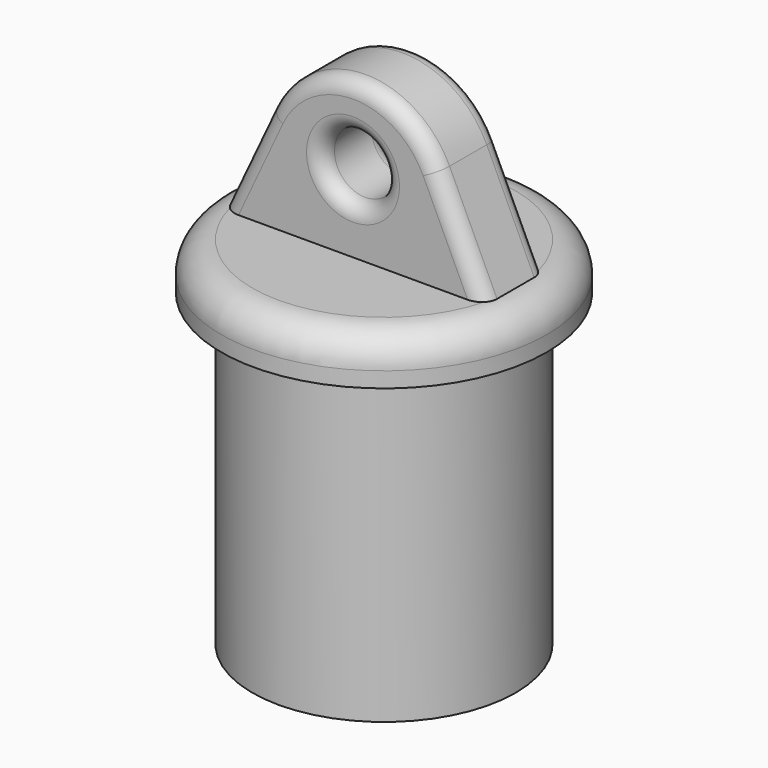
from build123d import *

# Parameters (mm, degrees)
F0_R          = 10.5
F1_DEPTH      = 3
F2_R          = 2
F3_R          = 7
F4_DEPTH      = 0.5
F5_W          = 1.5
F5_H          = 20
F7_R          = 2
F8_DEPTH      = 2.5
F8_DEPTH_BACK = 2.5
F9_T8_DEPTH   = 9.7284161474
F9_T13_DEPTH  = 9.7284161474
F9_T16_ANGLE  = 129.7914851202
F9_T20_DEPTH  = 9.7284161474
F9_T23_ANGLE  = 129.7914851202
F9_T27_DEPTH  = 9.7284161474


# Not quite as in the source:
# - a fillet or chamfer that OpenCascade refuses, or shapes differently, is made with other operations: its cross-section is extruded or revolved along the edge and cut away or added


with BuildPart() as f1:
    # F0 (on Top) → F1 (new body)
    with BuildSketch(Plane.XY):
        Circle(F0_R)
    extrude(amount=F1_DEPTH)

    # F2
    f2_edges = [f1.edges().sort_by_distance(p)[0] for p in [
        (-10.5, 0, 3),
    ]]
    fillet(f2_edges, radius=F2_R)

    # F3 (on face) → F4 (cut)
    with BuildSketch(Plane(origin=(0, 0, 0), x_dir=(1, 0, 0), z_dir=(0, 0, -1))):
        Circle(F3_R)
    extrude(amount=-F4_DEPTH, mode=Mode.SUBTRACT)

    # F5 (on Front) → F6 (revolve)
    with BuildSketch(Plane.XZ):
        with Locations((7.75, -10)):
            Rectangle(F5_W, F5_H)
    revolve(axis=Axis((0, 0, -11.0487695783), (0, 0, -1)))

    # F7 (on Front) → F8 (join, two sides)
    with BuildSketch(Plane.XZ) as f8_sk:
        with BuildLine():
            Line((-5.4332236548, 9.5456002665), (-8.5, 3))
            Line((-8.5, 3), (8.5, 3))
            Line((8.5, 3), (5.4332236548, 9.5456002665))
            ThreePointArc((5.4332236548, 9.5456002665), (0, 13), (-5.4332236548, 9.5456002665))
        make_face()
        with Locations((0, 8)):
            Circle(F7_R, mode=Mode.SUBTRACT)
    extrude(amount=F8_DEPTH)
    extrude(f8_sk.sketch, amount=-F8_DEPTH_BACK)

    # F9: fillet of radius 1 on 4 edges, made by hand

    # F9_s1 → F9_t2 (revolve, cut)
    with BuildSketch(Plane.XY.offset(8)):
        with BuildLine():
            ThreePointArc((3, 2.5), (2.2928932188, 2.2071067812), (2, 1.5))
            Line((2, 1.5), (2, 2.5))
            Line((2, 2.5), (3, 2.5))
        make_face()
    revolve(axis=Axis((0, 2.5, 8), (0, -1, 0)), mode=Mode.SUBTRACT)

    # F9_s3 → F9_t4 (revolve, cut)
    with BuildSketch(Plane.XY.offset(8)):
        with BuildLine():
            ThreePointArc((3, -2.5), (2.2928932188, -2.2071067812), (2, -1.5))
            Line((2, -1.5), (2, -2.5))
            Line((2, -2.5), (3, -2.5))
        make_face()
    revolve(axis=Axis((0, -2.5, 8), (0, -1, 0)), mode=Mode.SUBTRACT)


with BuildPart() as f9_tool6:
    # F9_s7 → F9_t8 (new body)
    with BuildSketch(Plane(origin=(1.4381178705, 0, -3.0694591509), x_dir=(0, 1, 0), z_dir=(-0.4242667111, 0, 0.9055372758))):
        with BuildLine():
            ThreePointArc((-1.5, -8.9698669776), (-2.2071067812, -8.6769737588), (-2.5, -7.9698669776))
            Line((-2.5, -7.9698669776), (-2.5, -8.9698669776))
            Line((-2.5, -8.9698669776), (-1.5, -8.9698669776))
        make_face()
    extrude(amount=F9_T8_DEPTH)

    split(bisect_by=Plane.XY.offset(3), keep=Keep.TOP)


with BuildPart() as f1_1:
    add(f1.part)

    # F9_t5: cut F9_tool6
    add(f9_tool6.part, mode=Mode.SUBTRACT)


with BuildPart() as f9_tool11:
    # F9_s12 → F9_t13 (new body)
    with BuildSketch(Plane(origin=(1.4381178705, 0, -3.0694591509), x_dir=(0, 1, 0), z_dir=(-0.4242667111, 0, 0.9055372758))):
        with BuildLine():
            ThreePointArc((2.5, -7.9698669776), (2.2071067812, -8.6769737588), (1.5, -8.9698669776))
            Line((1.5, -8.9698669776), (2.5, -8.9698669776))
            Line((2.5, -8.9698669776), (2.5, -7.9698669776))
        make_face()
    extrude(amount=F9_T13_DEPTH)

    split(bisect_by=Plane.XY.offset(3), keep=Keep.TOP)


with BuildPart() as f1_2:
    add(f1_1.part)

    # F9_t10: cut F9_tool11
    add(f9_tool11.part, mode=Mode.SUBTRACT)

    # F9_s15 → F9_t16 (revolve, cut)
    with BuildSketch(Plane(origin=(-2.6893252524, 0, 5.7399843051), x_dir=(0, 1, 0), z_dir=(0.4242667111, 0, -0.9055372758))):
        with BuildLine():
            ThreePointArc((2.5, 7.9698669776), (2.2071067812, 8.6769737588), (1.5, 8.9698669776))
            Line((1.5, 8.9698669776), (2.5, 8.9698669776))
            Line((2.5, 8.9698669776), (2.5, 7.9698669776))
        make_face()
    revolve(axis=Axis((0, 2.5, 7), (0, -1, 0)), revolution_arc=F9_T16_ANGLE, mode=Mode.SUBTRACT)


with BuildPart() as f9_tool18:
    # F9_s19 → F9_t20 (new body)
    with BuildSketch(Plane(origin=(2.6893252524, 0, 5.7399843051), x_dir=(0, 1, 0), z_dir=(-0.4242667111, 0, -0.9055372758))):
        with BuildLine():
            ThreePointArc((2.5, -7.9698669776), (2.2071067812, -8.6769737588), (1.5, -8.9698669776))
            Line((1.5, -8.9698669776), (2.5, -8.9698669776))
            Line((2.5, -8.9698669776), (2.5, -7.9698669776))
        make_face()
    extrude(amount=F9_T20_DEPTH)

    split(bisect_by=Plane.XY.offset(3), keep=Keep.TOP)


with BuildPart() as f1_3:
    add(f1_2.part)

    # F9_t17: cut F9_tool18
    add(f9_tool18.part, mode=Mode.SUBTRACT)

    # F9_s22 → F9_t23 (revolve, cut)
    with BuildSketch(Plane(origin=(-2.6893252524, 0, 5.7399843051), x_dir=(0, 1, 0), z_dir=(0.4242667111, 0, -0.9055372758))):
        with BuildLine():
            ThreePointArc((-2.5, 7.9698669776), (-2.2071067812, 8.6769737588), (-1.5, 8.9698669776))
            Line((-1.5, 8.9698669776), (-2.5, 8.9698669776))
            Line((-2.5, 8.9698669776), (-2.5, 7.9698669776))
        make_face()
    revolve(axis=Axis((0, -2.5, 7), (0, -1, 0)), revolution_arc=F9_T23_ANGLE, mode=Mode.SUBTRACT)


with BuildPart() as f9_tool25:
    # F9_s26 → F9_t27 (new body)
    with BuildSketch(Plane(origin=(2.6893252524, 0, 5.7399843051), x_dir=(0, 1, 0), z_dir=(-0.4242667111, 0, -0.9055372758))):
        with BuildLine():
            ThreePointArc((-1.5, -8.9698669776), (-2.2071067812, -8.6769737588), (-2.5, -7.9698669776))
            Line((-2.5, -7.9698669776), (-2.5, -8.9698669776))
            Line((-2.5, -8.9698669776), (-1.5, -8.9698669776))
        make_face()
    extrude(amount=F9_T27_DEPTH)

    split(bisect_by=Plane.XY.offset(3), keep=Keep.TOP)


with BuildPart() as f1_4:
    add(f1_3.part)

    # F9_t24: cut F9_tool25
    add(f9_tool25.part, mode=Mode.SUBTRACT)


solid = f1_4.part
